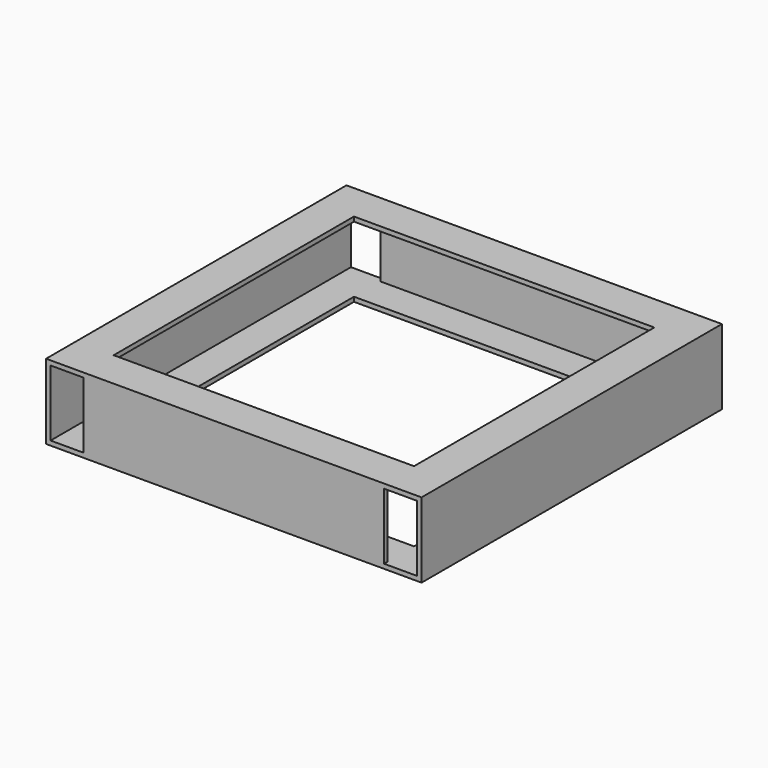
from build123d import *

# Parameters (mm, degrees)
F0_W      = 250
F0_H      = 250
F0_W_2    = 200
F0_H_2    = 200
F1_DEPTH  = 50
F2_W      = 22
F2_H      = 44
F3_DEPTH  = 250
F6_W      = 25
F6_H      = 44
F7_DEPTH  = 125
F8_DEPTH  = 25
F9_DEPTH  = 25
F12_DEPTH = 122
F13_DEPTH = 122


# Not quite as in the source:
# - an extrude ends at something that could not be found from the text; its depth is read off the source's solid
# - a feature of the source that left no trace in its solid (it failed there, or was rolled back) is left out


with BuildPart() as f1:
    # F0 (on Top) → F1 (new body)
    with BuildSketch(Plane.XY):
        Rectangle(F0_W, F0_H)
        Rectangle(F0_W_2, F0_H_2, mode=Mode.SUBTRACT)
    extrude(amount=F1_DEPTH)

    # F2 (on face) → F3 (cut, through all)
    with BuildSketch(Plane.XZ.offset(125)):
        with Locations((-111, 25)):
            Rectangle(F2_W, F2_H)
        with Locations((111, 25)):
            Rectangle(F2_W, F2_H)
    extrude(amount=-F3_DEPTH, mode=Mode.SUBTRACT)

    # F6 (on Right) → F7 (cut, through all)
    with BuildSketch(Plane.YZ):
        with Locations((109.5, 25)):
            Rectangle(F6_W, F6_H)
        with Locations((-109.5, 25)):
            Rectangle(F6_W, F6_H)
    extrude(amount=-F7_DEPTH, mode=Mode.SUBTRACT)

    # F8 (add): a face of the model
    f8_faces = [f1.faces().sort_by_distance(p)[0] for p in [
        (-123.5, 97, 25),
    ]]
    extrude(f8_faces, amount=F8_DEPTH)

    # F9 (add): a face of the model
    f9_faces = [f1.faces().sort_by_distance(p)[0] for p in [
        (-123.5, -122, 25),
    ]]
    extrude(f9_faces, amount=F9_DEPTH)

    # F12 (cut, through all): a face of the model
    f12_faces = [f1.faces().sort_by_distance(p)[0] for p in [
        (0, -111, 25),
    ]]
    extrude(f12_faces, amount=-F12_DEPTH, mode=Mode.SUBTRACT)

    # F13 (cut, through all): a face of the model
    f13_faces = [f1.faces().sort_by_distance(p)[0] for p in [
        (0, 111, 25),
    ]]
    extrude(f13_faces, amount=-F13_DEPTH, mode=Mode.SUBTRACT)


solid = f1.part
